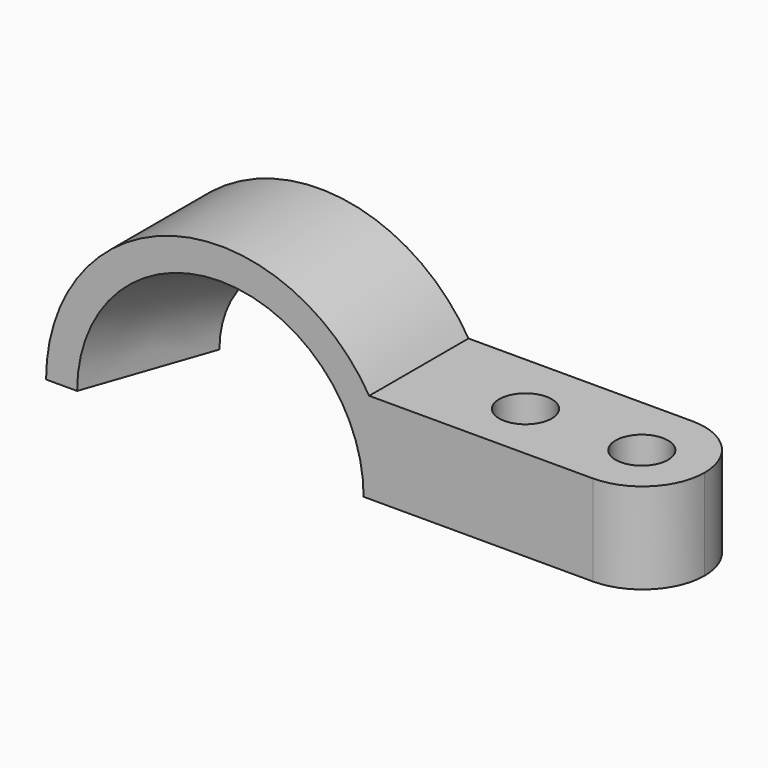
from build123d import *

# Parameters (mm, degrees)
F1_DEPTH = 52
F5_R     = 11
F6_DEPTH = 50
F7_R     = 25.99999


# Not quite as in the source:
# - a fillet or chamfer is up to 0.001 mm smaller than in the source, because OpenCascade refuses the exact size


with BuildPart() as f1:
    # F0 (on Front) → F1 (new body)
    with BuildSketch(Plane.XZ):
        with BuildLine():
            ThreePointArc((-42, 0), (0, 42), (42, 0))
            Line((42, 0), (73, 0))
            Line((73, 0), (182, 0))
            Line((182, 0), (182, 38))
            Line((182, 38), (62.329768169, 38))
            ThreePointArc((62.329768169, 38), (-19.7348286497, 70.2818364741), (-73, 0))
            Line((-73, 0), (-42, 0))
        make_face()
    extrude(amount=F1_DEPTH)

    # F2 (on face) → F3 (revolve, cut)
    with BuildSketch(Plane(origin=(0, 0, 0), x_dir=(1, 0, 0), z_dir=(0, 0, -1))):
        Polygon((-42, 52), (-60, 52), (-42, 0), align=None)
    revolve(axis=Axis((0, -26.5927761793, 0), (0, 1, 0)), mode=Mode.SUBTRACT)

    # F5 (on face) → F6 (cut)
    with BuildSketch(Plane(origin=(0, 0, 0), x_dir=(1, 0, 0), z_dir=(0, 0, -1))):
        with Locations((156, 26.3603460044)):
            Circle(F5_R)
        with Locations((108, 27.2682987475)):
            Circle(F5_R)
    extrude(amount=-F6_DEPTH, mode=Mode.SUBTRACT)

    # F7 (radius 26 in the source; OpenCascade refuses exactly that, so slightly less here)
    f7_edges = [f1.edges().sort_by_distance(p)[0] for p in [
        (182, -52, 19),
        (182, 0, 19),
    ]]
    fillet(f7_edges, radius=F7_R)


solid = f1.part
